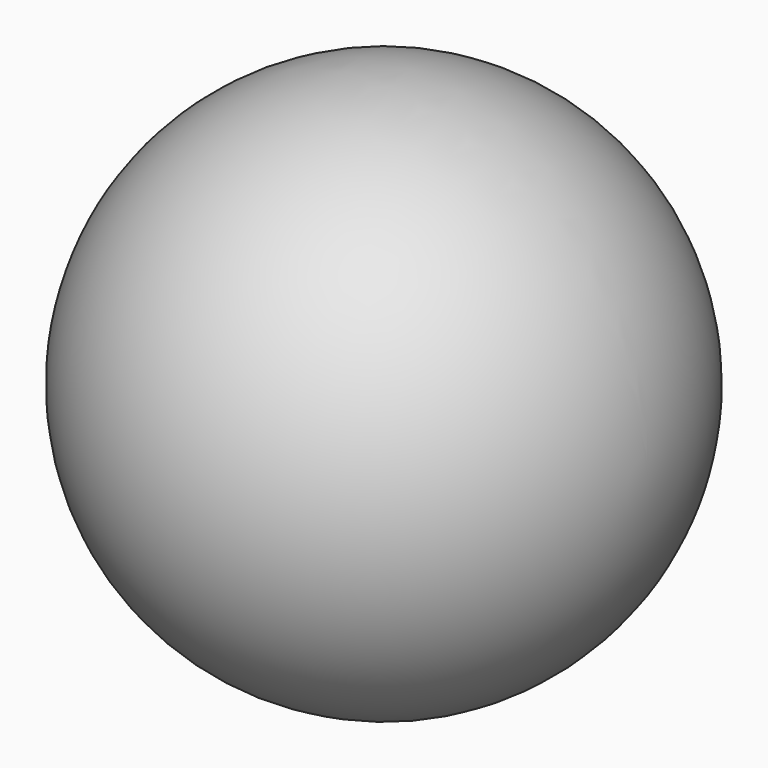
from build123d import *


# Not quite as in the source:
# - a fillet or chamfer that OpenCascade refuses, or shapes differently, is made with other operations: its cross-section is extruded or revolved along the edge and cut away or added


with BuildPart() as f1:
    # F0 (on Front) → F1 (revolve)
    with BuildSketch(Plane.XZ):
        with BuildLine():
            Line((7.62, 0), (12.407513929, 0))
            ThreePointArc((12.407513929, 0), (7.7010148654, 6.1336289969), (0.558252615, 3.175))
            Line((0.558252615, 3.175), (0.558252615, 1.905))
            Line((0.558252615, 1.905), (7.62, 1.905))
            Line((7.62, 1.905), (7.62, 0))
        make_face()
    revolve(axis=Axis((8.8458018737, 0, 0), (1, 0, 0)))

    # F2: chamfer of 0.254 on 3 edges, made by hand

    # F2_s1 → F2_t2 (revolve)
    with BuildSketch(Plane.XZ):
        Polygon((7.366, 1.905), (7.62, 1.651), (7.62, 1.905), align=None)
    revolve(axis=Axis((7.62, 0, 0), (1, 0, 0)))

    # F2_s3 → F2_t4 (revolve, cut)
    with BuildSketch(Plane.XZ):
        with BuildLine():
            Line((0.558252615, 3.1061953814), (0.5937000602, 3.235620189))
            ThreePointArc((0.5937000602, 3.235620189), (0.5783706102, 3.2095931974), (0.558252615, 3.175))
            Line((0.558252615, 3.175), (0.558252615, 3.1061953814))
        make_face()
    revolve(axis=Axis((0.558252615, 0, 0), (1, 0, 0)), mode=Mode.SUBTRACT)

    # F2_s5 → F2_t6 (revolve, cut)
    with BuildSketch(Plane.XZ):
        Polygon((0.558252615, 2.159), (0.812252615, 1.905), (0.558252615, 1.905), align=None)
    revolve(axis=Axis((0.558252615, 0, 0), (1, 0, 0)), mode=Mode.SUBTRACT)


solid = f1.part
